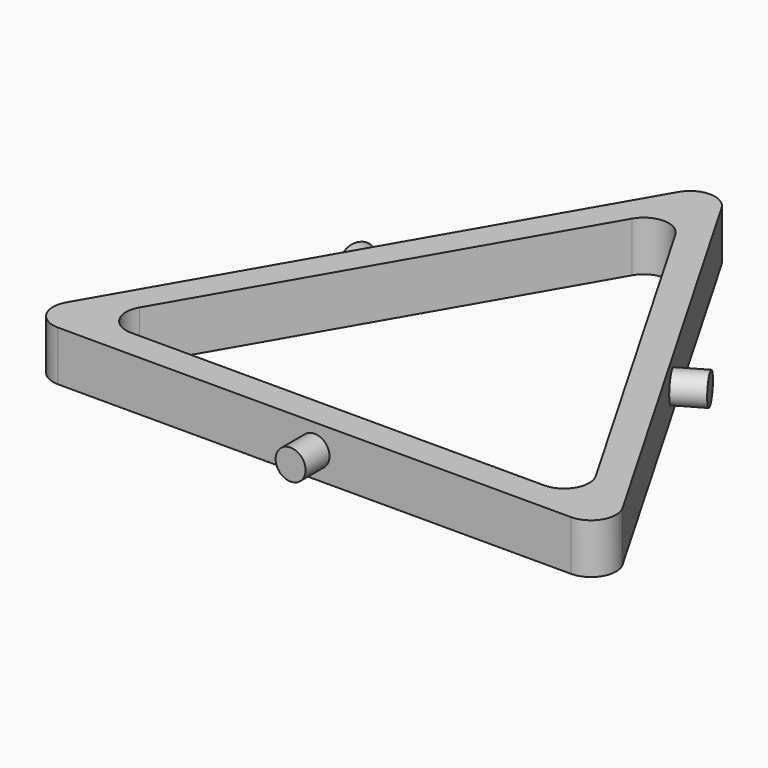
from build123d import *

# Parameters (mm, degrees)
F1_DEPTH        = 10
F2_R            = 5
F3_R            = 3
F4_DEPTH        = 6
F4_COPIES_COUNT = 3


# Not quite as in the source:
# - a pattern or mirror of a feature is missing from the dataset's text; its kind, count and spacing are read off the source's solid


with BuildPart() as f1:
    # F0 (on Top) → F1 (new body)
    with BuildSketch(Plane.XY):
        Polygon((60, -34.6410161514), (0, 69.2820323028), (-60, -34.6410161514), align=None)
        Polygon((0, 57.735026919), (50, -28.8675134595), (-50, -28.8675134595), align=None, mode=Mode.SUBTRACT)
    extrude(amount=F1_DEPTH)

    # F2
    f2_edges = [f1.edges().sort_by_distance(p)[0] for p in [
        (-60, -34.641016, 5),
        (60, -34.641016, 5),
        (0, 69.282032, 5),
        (50, -28.867513, 5),
        (0, 57.735027, 5),
        (-50, -28.867513, 5),
    ]]
    fillet(f2_edges, radius=F2_R)

    # F3 (on face) → F4 (join)
    with BuildSketch(Plane.XZ.offset(34.6410161514)):
        with Locations((0, 5)):
            Circle(F3_R)
    f4 = extrude(amount=F4_DEPTH)

    # F4_copies: F4 ×3 about axis
    f4_copies_axis = Axis((0, 0, 0), (0, 0, 1))
    for i in range(1, F4_COPIES_COUNT):
        add(f4.rotate(f4_copies_axis, i * 360 / F4_COPIES_COUNT))


solid = f1.part
